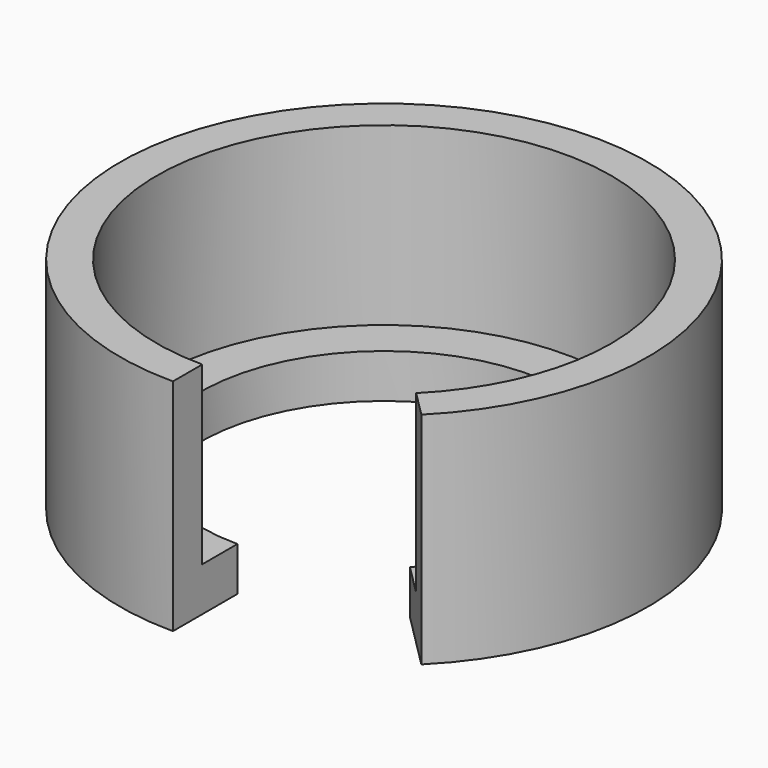
from build123d import *

# Parameters (mm, degrees)
F1_DEPTH = 3
F2_DEPTH = 15


with BuildPart() as f1:
    # F0 (on Top) → F1 (new body)
    with BuildSketch(Plane.XY):
        with BuildLine():
            ThreePointArc((0, -12.5), (-8.8388347648, 8.8388347648), (12.5, 0))
            ThreePointArc((12.5, 0), (11.5484941564, -4.7835429046), (8.8388347648, -8.8388347648))
            Line((8.8388347648, -8.8388347648), (10.9601551084, -10.9601551084))
            ThreePointArc((10.9601551084, -10.9601551084), (14.3201327539, -5.9315932017), (15.5, 0))
            ThreePointArc((15.5, 0), (-10.9601551084, 10.9601551084), (0, -15.5))
            Line((0, -15.5), (0, -12.5))
        make_face()
    extrude(amount=F1_DEPTH)

    # F0 (on Top) → F2 (join)
    with BuildSketch(Plane.XY):
        with BuildLine():
            Line((0, -18), (0, -15.5))
            ThreePointArc((0, -15.5), (-10.9601551084, 10.9601551084), (15.5, 0))
            ThreePointArc((15.5, 0), (14.3201327539, -5.9315932017), (10.9601551084, -10.9601551084))
            Line((10.9601551084, -10.9601551084), (12.7279220614, -12.7279220614))
            ThreePointArc((12.7279220614, -12.7279220614), (16.6298315852, -6.8883017826), (18, 0))
            ThreePointArc((18, 0), (-12.7279220614, 12.7279220614), (0, -18))
        make_face()
    extrude(amount=F2_DEPTH)


solid = f1.part
